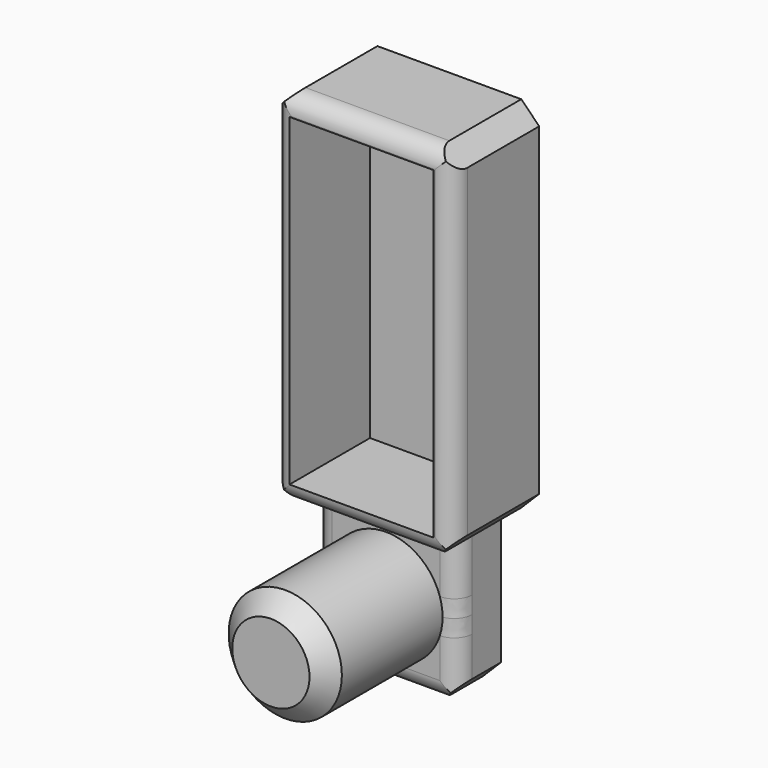
from build123d import *

# Parameters (mm, degrees)
F1_W         = 50
F1_H         = 100
F2_DEPTH     = 30
F4_W         = 40
F4_H         = 90
F5_DEPTH     = 28
F6_SIZE      = 5
F7_T1_DEPTH  = 115
F7_T3_DEPTH  = 65
F8_W         = 40
F8_H         = 20
F9_DEPTH     = 40
F10_R        = 15.7450666382
F11_DEPTH    = 40
F12_R        = 5
F13_T1_DEPTH = 6.3508529611
F13_T3_DEPTH = 6.3508529611
F13_T5_DEPTH = 40.7168298797
F13_T7_DEPTH = 65.7168298797
F13_T9_DEPTH = 52.8584149398


# Not quite as in the source:
# - a fillet or chamfer that OpenCascade refuses, or shapes differently, is made with other operations: its cross-section is extruded or revolved along the edge and cut away or added


with BuildPart() as f2:
    # F1 (on face) → F2 (new body)
    with BuildSketch(Plane.XZ):
        Rectangle(F1_W, F1_H)
    extrude(amount=F2_DEPTH)

    # F4 (on face) → F5 (cut)
    with BuildSketch(Plane.XZ.offset(30)):
        with Locations((-0.4633623362, -0.2909506857)):
            Rectangle(F4_W, F4_H)
    extrude(amount=-F5_DEPTH, mode=Mode.SUBTRACT)

    # F6
    f6_edges = [f2.edges().sort_by_distance(p)[0] for p in [
        (25, -15, 50),
        (-25, -15, 50),
        (-25, -15, -50),
        (25, -15, -50),
    ]]
    chamfer(f6_edges, length=F6_SIZE)

    # F7: fillet of radius 5 on 4 edges, made by hand

    # F7_s2 → F7_t1 (cut)
    with BuildSketch(Plane.XY.offset(-57.5)):
        with BuildLine():
            ThreePointArc((-20, -30), (-23.5355339059, -28.5355339059), (-25, -25))
            Line((-25, -25), (-25, -30))
            Line((-25, -30), (-20, -30))
        make_face()
        with BuildLine():
            ThreePointArc((20, -30), (23.5355339059, -28.5355339059), (25, -25))
            Line((25, -25), (25, -30))
            Line((25, -30), (20, -30))
        make_face()
    extrude(amount=F7_T1_DEPTH, mode=Mode.SUBTRACT)

    # F7_s4 → F7_t3 (cut)
    with BuildSketch(Plane.YZ.offset(-32.5)):
        with BuildLine():
            ThreePointArc((-30, 45), (-28.5355339059, 48.5355339059), (-25, 50))
            Line((-25, 50), (-30, 50))
            Line((-30, 50), (-30, 45))
        make_face()
        with BuildLine():
            ThreePointArc((-25, -50), (-28.5355339059, -48.5355339059), (-30, -45))
            Line((-30, -45), (-30, -50))
            Line((-30, -50), (-25, -50))
        make_face()
    extrude(amount=F7_T3_DEPTH, mode=Mode.SUBTRACT)

    # F8 (on face) → F9 (join)
    with BuildSketch(Plane(origin=(0, 0, -50), x_dir=(1, 0, 0), z_dir=(0, 0, -1))):
        with Locations((0, 12.041676566)):
            Rectangle(F8_W, F8_H)
    extrude(amount=F9_DEPTH)

    # F10 (on face) → F11 (join)
    with BuildSketch(Plane.XZ.offset(22.041676566)):
        with Locations((0, -69.2195519805)):
            Circle(F10_R)
    extrude(amount=F11_DEPTH)

    # F12
    f12_edges = [f2.edges().sort_by_distance(p)[0] for p in [
        (-20, -22.041677, -70),
        (20, -22.041677, -70),
        (0, -22.041677, -90),
    ]]
    fillet(f12_edges, radius=F12_R)

    # F13: chamfer of 5 on 7 edges, made by hand

    # F13_s2 → F13_t1 (cut)
    with BuildSketch(Plane(origin=(-32.652774478, 32.652774478, -32.652774478), x_dir=(-0.7071067812, -0.7071067812, 0), z_dir=(-0.5773502692, 0.5773502692, -0.5773502692))):
        Polygon((12.0502850626, -64.1119959897), (19.1213528745, -64.1119959897), (15.5858189685, -70.2357203466), align=None)
    extrude(amount=F13_T1_DEPTH, mode=Mode.SUBTRACT)

    # F13_s4 → F13_t3 (cut)
    with BuildSketch(Plane(origin=(32.652774478, 32.652774478, -32.652774478), x_dir=(-0.7071067812, 0.7071067812, 0), z_dir=(0.5773502692, 0.5773502692, -0.5773502692))):
        Polygon((-19.1213528745, -64.1119959897), (-15.5858189685, -70.2357203466), (-12.0502850626, -64.1119959897), align=None)
    extrude(amount=F13_T3_DEPTH, mode=Mode.SUBTRACT)

    # F13_s6 → F13_t5 (cut)
    with BuildSketch(Plane.XZ.offset(-10.8167383738)):
        Polygon((-15, -90), (-20, -85), (-20, -90), align=None)
        Polygon((20, -85), (15, -90), (20, -90), align=None)
    extrude(amount=F13_T5_DEPTH, mode=Mode.SUBTRACT)

    # F13_s8 → F13_t7 (cut)
    with BuildSketch(Plane.YZ.offset(-32.8584149398)):
        Polygon((-2.041676566, -85), (-7.041676566, -90), (-2.041676566, -90), align=None)
    extrude(amount=F13_T7_DEPTH, mode=Mode.SUBTRACT)

    # F13_s10 → F13_t9 (cut)
    with BuildSketch(Plane.XY.offset(-102.8584149398)):
        Polygon((20, -7.041676566), (15, -2.041676566), (20, -2.041676566), align=None)
        Polygon((-15, -2.041676566), (-20, -7.041676566), (-20, -2.041676566), align=None)
    extrude(amount=F13_T9_DEPTH, mode=Mode.SUBTRACT)

    # F13_s11 → F13_t12 (revolve, cut)
    with BuildSketch(Plane.XY.offset(-69.2195519805)):
        Polygon((15.7450666382, -57.041676566), (10.7450666382, -62.041676566), (15.7450666382, -62.041676566), align=None)
    revolve(axis=Axis((0, -62.041676566, -69.2195519805), (0, -1, 0)), mode=Mode.SUBTRACT)


solid = f2.part
